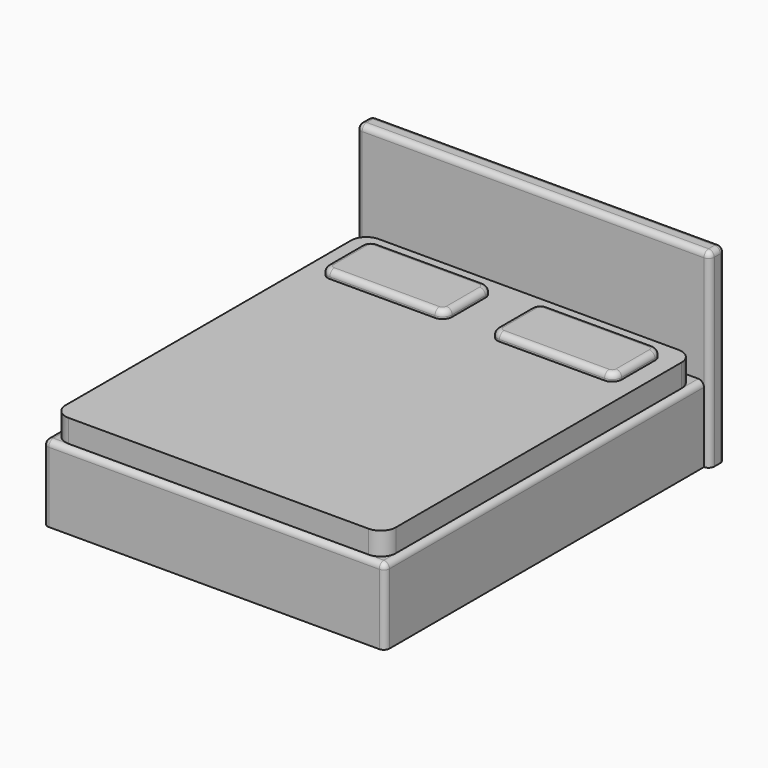
from build123d import *

# Parameters (mm, degrees)
F0_W     = 180
F0_H     = 210
F1_DEPTH = 40
F2_W     = 186
F2_H     = 10
F3_DEPTH = 100
F4_W     = 174
F4_H     = 204
F5_DEPTH = 12
F6_W     = 65.3649838641
F6_H     = 31.9020412862
F7_DEPTH = 4
F8_DEPTH = 4
F9_R     = 8
F10_R    = 3
F11_R    = 2.99999
F12_R    = 5
F13_R    = 3


# Not quite as in the source:
# - a fillet or chamfer is up to 0.001 mm smaller than in the source, because OpenCascade refuses the exact size


with BuildPart() as f1:
    # F0 (on Top) → F1 (new body)
    with BuildSketch(Plane.XY):
        Rectangle(F0_W, F0_H)
    extrude(amount=F1_DEPTH)

    # F2 (on Top) → F3 (join)
    with BuildSketch(Plane.XY):
        with Locations((0, 110)):
            Rectangle(F2_W, F2_H)
    extrude(amount=F3_DEPTH)

    # F4 (on face) → F5 (join)
    with BuildSketch(Plane.XY.offset(40)):
        Rectangle(F4_W, F4_H)
    extrude(amount=F5_DEPTH)

    # F6 (on face) → F7 (join)
    with BuildSketch(Plane.XY.offset(52)):
        with Locations((-44.6581854485, 77.6125434786)):
            Rectangle(F6_W, F6_H)
    extrude(amount=F7_DEPTH)

    # F6 (on face) → F8 (join)
    with BuildSketch(Plane.XY.offset(52)):
        with Locations((-44.6581854485, 77.6125434786)):
            Rectangle(F6_W, F6_H)
        with Locations((44.6581854485, 77.6125434786)):
            Rectangle(F6_W, F6_H)
    extrude(amount=F8_DEPTH)

    # F9
    f9_edges = [f1.edges().sort_by_distance(p)[0] for p in [
        (-87, -102, 46),
        (87, -102, 46),
        (87, 102, 46),
        (-87, 102, 46),
    ]]
    fillet(f9_edges, radius=F9_R)

    # F10
    f10_edges = [f1.edges().sort_by_distance(p)[0] for p in [
        (-93, 110, 100),
        (-93, 105, 50),
        (0, 105, 100),
        (93, 105, 50),
        (93, 110, 100),
        (0, 115, 100),
        (-93, 115, 50),
        (93, 115, 50),
    ]]
    fillet(f10_edges, radius=F10_R)

    # F11 (radius 3 in the source; OpenCascade refuses exactly that, so slightly less here)
    f11_edges = [f1.edges().sort_by_distance(p)[0] for p in [
        (-90, 0, 40),
        (0, -105, 40),
        (-90, -105, 20),
        (90, -105, 20),
        (90, 0, 40),
    ]]
    fillet(f11_edges, radius=F11_R)

    # F12
    f12_edges = [f1.edges().sort_by_distance(p)[0] for p in [
        (-77.340677, 61.661523, 54),
        (-11.975694, 61.661523, 54),
        (-11.975694, 93.563564, 54),
        (-77.340677, 93.563564, 54),
        (11.975694, 93.563564, 54),
        (11.975694, 61.661523, 54),
        (77.340677, 61.661523, 54),
        (77.340677, 93.563564, 54),
    ]]
    fillet(f12_edges, radius=F12_R)

    # F13
    f13_edges = [f1.edges().sort_by_distance(p)[0] for p in [
        (77.340677, 77.612543, 56),
        (75.876211, 63.125989, 56),
        (75.876211, 92.099098, 56),
        (44.658185, 61.661523, 56),
        (44.658185, 93.563564, 56),
        (13.44016, 63.125989, 56),
        (13.44016, 92.099098, 56),
        (11.975694, 77.612543, 56),
        (-44.658185, 93.563564, 56),
        (-13.44016, 92.099098, 56),
        (-75.876211, 92.099098, 56),
        (-11.975694, 77.612543, 56),
        (-77.340677, 77.612543, 56),
        (-13.44016, 63.125989, 56),
        (-75.876211, 63.125989, 56),
        (-44.658185, 61.661523, 56),
    ]]
    fillet(f13_edges, radius=F13_R)


solid = f1.part
